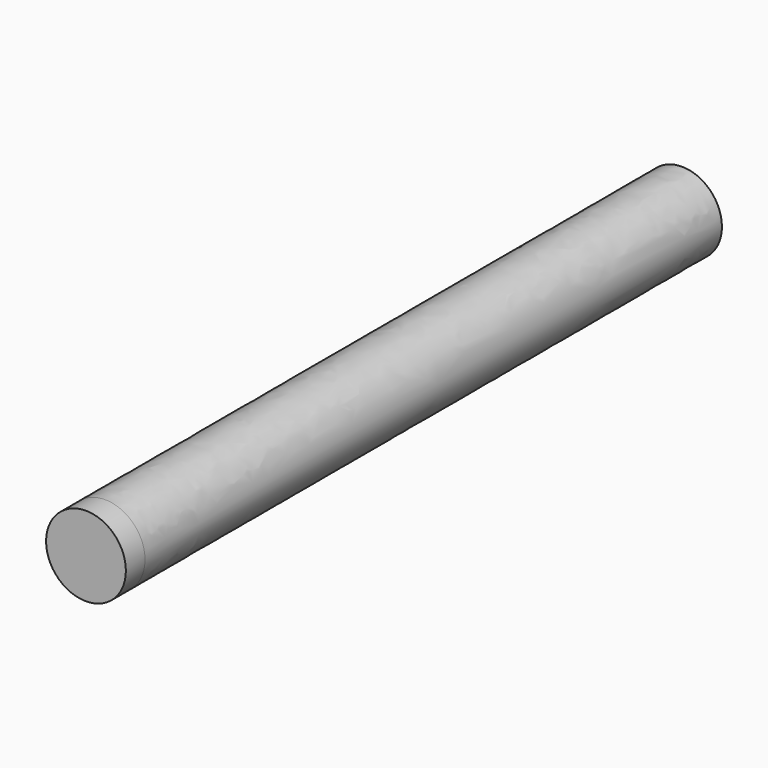
from build123d import *

# Parameters (mm, degrees)
F0_R = 5


# Not quite as in the source:
# - a feature of the source that left no trace in its solid (it failed there, or was rolled back) is left out
# - a pattern or mirror of a feature is missing from the dataset's text; its kind, count and spacing are read off the source's solid


with BuildPart() as f2:
    # F2: sweep along a path in F1
    with BuildLine(Plane.YZ) as f2_path:
        add(Plane.YZ * Edge.make_bspline(
            [(0, 0), (-10.4992447827, 0), (-42.2072799112, 0), (-81.3958233683, 0), (-90.3834476083, 0)],
            knots=[0, 0, 0, 0, 0.4898580308, 1, 1, 1, 1], degree=3))
    # F0 (on Front) → F2 (sweep)
    with BuildSketch(Plane.XZ):
        Circle(F0_R)
    sweep(path=f2_path.line)

    # F2_copies: F2 across plane


with BuildPart() as f2_1:
    add(f2.part)
    add(f2.part.mirror(Plane(origin=(0, -46.691724, 0), x_dir=(0, 0, -1), z_dir=(0, -1, 0))))


solid = f2_1.part
